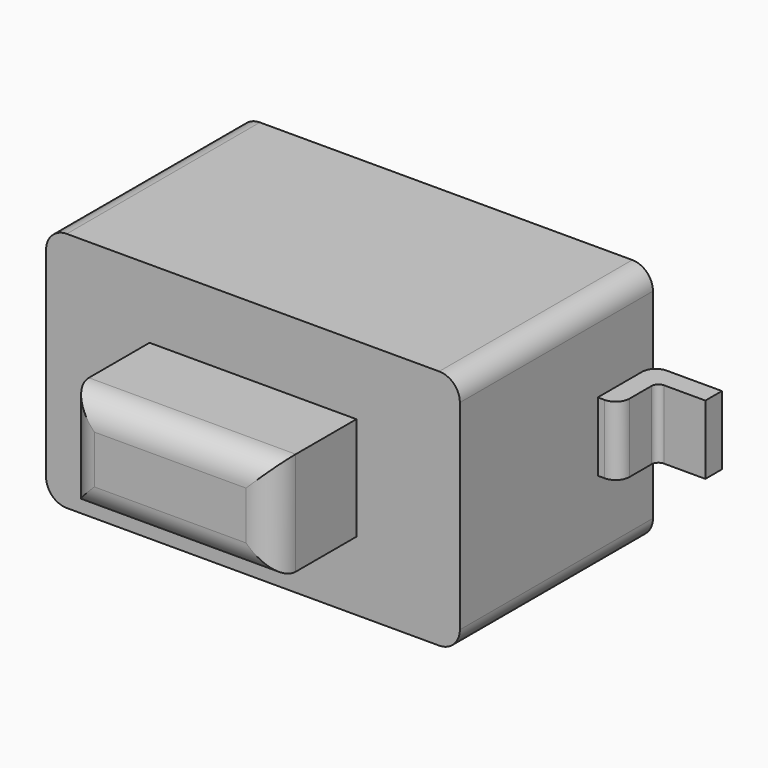
from build123d import *

# Parameters (mm, degrees)
F0_W     = 6
F0_H     = 3.5
F1_DEPTH = 3.5
F2_W     = 3
F2_H     = 1.5
F3_DEPTH = 1.5
F4_R     = 0.3
F5_R     = 0.4
F8_DEPTH = 0.5


# Not quite as in the source:
# - a pattern or mirror of a feature is missing from the dataset's text; its kind, count and spacing are read off the source's solid


with BuildPart() as f1:
    # F0 (on Front) → F1 (new body)
    with BuildSketch(Plane.XZ):
        with Locations((3, 1.75)):
            Rectangle(F0_W, F0_H)
    extrude(amount=F1_DEPTH)

    # F2 (on face) → F3 (join)
    with BuildSketch(Plane.XZ.offset(3.5)):
        with Locations((3, 1.75)):
            Rectangle(F2_W, F2_H)
    extrude(amount=F3_DEPTH)

    # F4
    f4_edges = [f1.edges().sort_by_distance(p)[0] for p in [
        (0, -1.75, 0),
        (0, -1.75, 3.5),
        (6, -1.75, 0),
        (6, -1.75, 3.5),
    ]]
    fillet(f4_edges, radius=F4_R)

    # F5
    f5_edges = [f1.edges().sort_by_distance(p)[0] for p in [
        (1.5, -5, 1.75),
        (3, -5, 2.5),
        (3, -5, 1),
        (4.5, -5, 1.75),
    ]]
    fillet(f5_edges, radius=F5_R)

    # F7 (on mid) → F8 (join, symmetric)
    with BuildSketch(Plane.XY.offset(1.75)):
        with BuildLine():
            Line((-0.1, -1), (0, -1))
            Line((0, -1), (0, -0.2))
            ThreePointArc((0, -0.2), (-0.0585786438, -0.0585786438), (-0.2, 0))
            Line((-0.2, 0), (-1, 0))
            Line((-1, 0), (-1, -0.3))
            Line((-1, -0.3), (-0.4, -0.3))
            ThreePointArc((-0.4, -0.3), (-0.3292893219, -0.3292893219), (-0.3, -0.4))
            Line((-0.3, -0.4), (-0.3, -0.8))
            ThreePointArc((-0.3, -0.8), (-0.2414213562, -0.9414213562), (-0.1, -1))
        make_face()
    f8 = extrude(amount=F8_DEPTH, both=True)

    # F8_copies: F8 across plane
    add(f8.mirror(Plane(origin=(3, 0, 0), x_dir=(0, 0, 1), z_dir=(1, 0, 0))))


solid = f1.part
